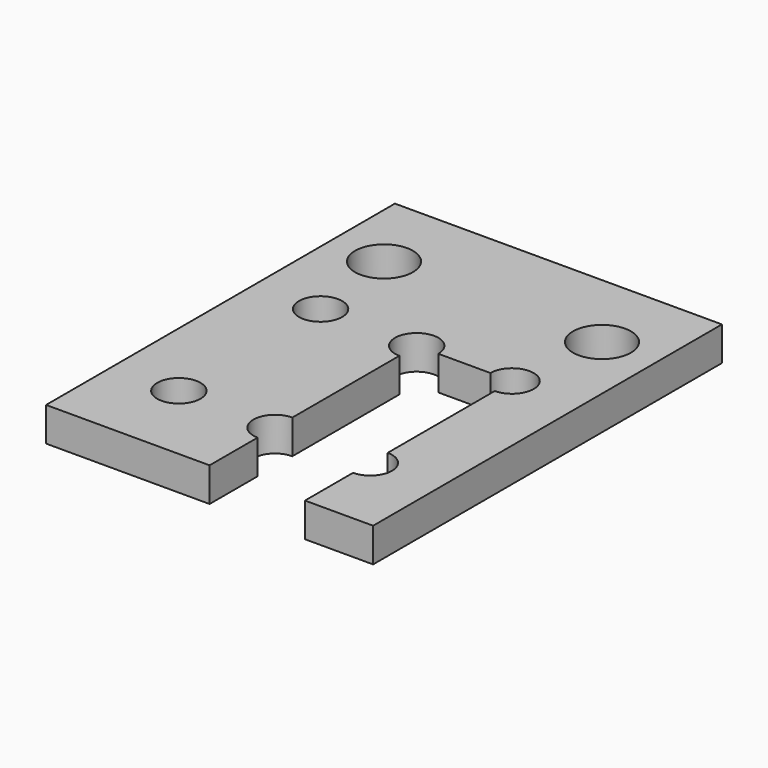
from build123d import *

# Parameters (mm, degrees)
F0_W     = 12.7
F0_H     = 19.05
F1_DEPTH = 7.9375
F2_D     = 10.0838
F3_D     = 13.49248


# Not quite as in the source:
# - a feature names something its author has since deleted; it is built from what else it names


with BuildPart() as f1:
    # F0 (on Top) → F1 (new body)
    with BuildSketch(Plane.XY):
        Polygon((25.5451762405, 40.8851695299), (-25.2548237595, 40.8851695299), (-25.2548237595, 21.8351695299), (-37.9548237595, 21.8351695299), (-37.9548237595, -60.7148304701), (0.1451762405, -60.7148304701), (0.1451762405, -41.6648304701), (0.1451762405, -0.3898304701), (22.3701762405, -0.3898304701), (22.3701762405, -41.6648304701), (22.3701762405, -60.7148304701), (38.2451762405, -60.7148304701), (38.2451762405, 21.8351695299), (25.5451762405, 21.8351695299), align=None)
        with Locations((-31.6048237595, 31.3601695299)):
            Rectangle(F0_W, F0_H)
        with Locations((31.8951762405, 31.3601695299)):
            Rectangle(F0_W, F0_H)
    extrude(amount=F1_DEPTH)

    # F2 (through all)
    with Locations(Plane(origin=(0, 0, 0), x_dir=(1, 0, 0), z_dir=(0, 0, -1))):
        with Locations((0.1451762405, 0.3898304701), (0.1451762405, 41.6648304701), (-22.5665104002, 0), (-22.5665104002, 41.275), (22.3701762405, 41.6648304701), (22.3701762405, 0.3898304701)):
            Hole(F2_D / 2)

    # F3 (through all)
    with Locations(Plane(origin=(0, 0, 0), x_dir=(1, 0, 0), z_dir=(0, 0, -1))):
        with Locations((-25.2548237595, -21.8351695299), (25.5451762405, -21.8351695299)):
            Hole(F3_D / 2)


solid = f1.part
